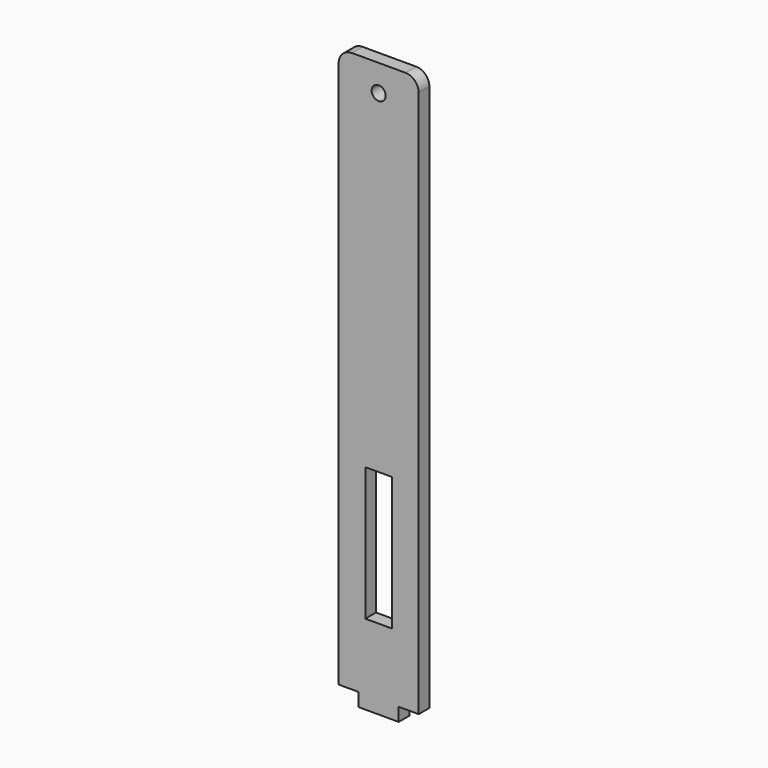
from build123d import *

# Parameters (mm, degrees)
F0_W     = 15
F0_H     = 5
F1_DEPTH = 2.5
F3_D     = 5.25
F4_R     = 5
F5_W     = 10
F5_H     = 50
F6_DEPTH = 10


with BuildPart() as f1:
    # F0 (on Front) → F1 (new body, symmetric)
    with BuildSketch(Plane.XZ):
        Polygon((15, -105), (15, 105), (-15, 105), (-15, -105), (-7.5, -105), (-7.5, -100), (7.5, -100), (7.5, -105), align=None)
        with Locations((0, -107.5)):
            Rectangle(F0_W, F0_H)
        with Locations((0, -102.5)):
            Rectangle(F0_W, F0_H)
    extrude(amount=F1_DEPTH, both=True)

    # F3 (through all)
    with Locations(Plane.XZ.offset(2.5)):
        with Locations((0, 95)):
            Hole(F3_D / 2)

    # F4
    f4_edges = [f1.edges().sort_by_distance(p)[0] for p in [
        (15, 0, 105),
        (-15, 0, 105),
    ]]
    fillet(f4_edges, radius=F4_R)

    # F5 (on face) → F6 (cut)
    with BuildSketch(Plane.XZ.offset(2.5)):
        with Locations((0, -55)):
            Rectangle(F5_W, F5_H)
    extrude(amount=-F6_DEPTH, mode=Mode.SUBTRACT)


solid = f1.part
